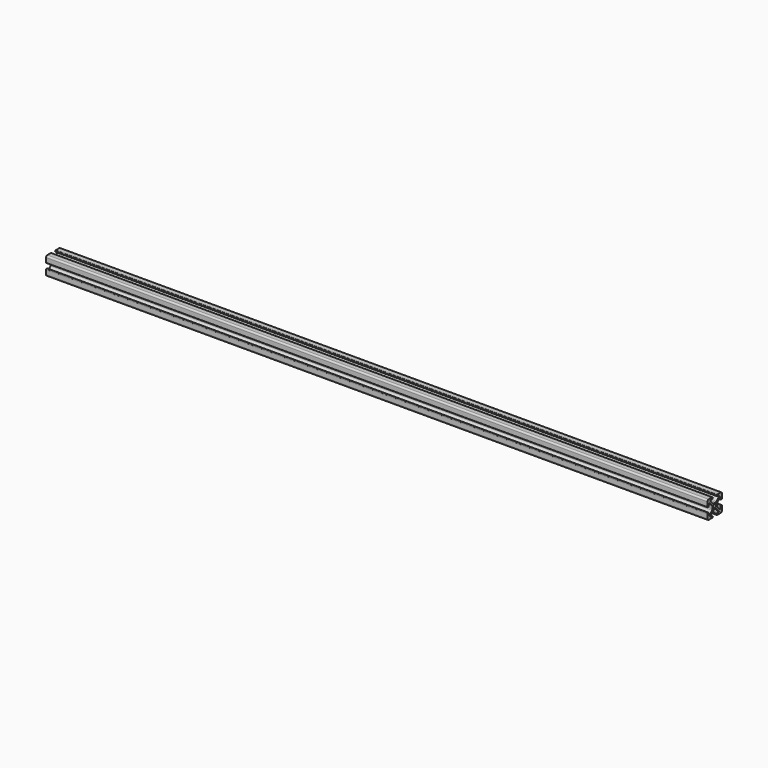
from build123d import *

# Parameters (mm, degrees)
F0_R     = 2.5
F2_DEPTH = 914.4
F3_R     = 2.14
F4_R     = 1.06999


# Not quite as in the source:
# - a fillet or chamfer is up to 0.001 mm smaller than in the source, because OpenCascade refuses the exact size


with BuildPart() as f2:
    # F0 (on Right) → F2 (new body)
    with BuildSketch(Plane.YZ):
        Polygon((2.5367914883, -4.05), (4.05, -4.05), (4.05, -2.5367914883), (4.05, 2.5367914883), (4.05, 4.05), (2.5367914883, 4.05), (-2.5367914883, 4.05), (-4.05, 4.05), (-4.05, 2.5367914883), (-4.05, -2.5367914883), (-4.05, -4.05), (-2.5367914883, -4.05), align=None)
        Circle(F0_R, mode=Mode.SUBTRACT)
        Polygon((-10.36, 8.8467914883), (-4.05, 2.5367914883), (-4.05, 4.05), (-2.5367914883, 4.05), (-8.8467914883, 10.36), (-3.25, 10.36), (-3.25, 12.5), (-12.5, 12.5), (-12.5, 3.25), (-10.36, 3.25), align=None)
        Polygon((4.05, 4.05), (4.05, 2.5367914883), (10.36, 8.8467914883), (10.36, 3.25), (12.5, 3.25), (12.5, 12.5), (3.25, 12.5), (3.25, 10.36), (8.8467914883, 10.36), (2.5367914883, 4.05), align=None)
        Polygon((-8.8467914883, -10.36), (-2.5367914883, -4.05), (-4.05, -4.05), (-4.05, -2.5367914883), (-10.36, -8.8467914883), (-10.36, -3.25), (-12.5, -3.25), (-12.5, -12.5), (-3.25, -12.5), (-3.25, -10.36), align=None)
        Polygon((4.05, -2.5367914883), (4.05, -4.05), (2.5367914883, -4.05), (8.8467914883, -10.36), (3.25, -10.36), (3.25, -12.5), (12.5, -12.5), (12.5, -3.25), (10.36, -3.25), (10.36, -8.8467914883), align=None)
    extrude(amount=F2_DEPTH)

    # F3
    f3_edges = [f2.edges().sort_by_distance(p)[0] for p in [
        (457.2, -12.5, 12.5),
        (457.2, 12.5, 12.5),
        (457.2, 12.5, -12.5),
        (457.2, -12.5, -12.5),
        (457.2, -4.05, 2.536791),
        (457.2, -4.05, -2.536791),
        (457.2, -2.536791, 4.05),
        (457.2, 2.536791, 4.05),
        (457.2, 4.05, 2.536791),
        (457.2, 4.05, -2.536791),
        (457.2, -2.536791, -4.05),
        (457.2, 2.536791, -4.05),
    ]]
    fillet(f3_edges, radius=F3_R)

    # F4 (radius 1.07 in the source; OpenCascade refuses exactly that, so slightly less here)
    f4_edges = [f2.edges().sort_by_distance(p)[0] for p in [
        (457.2, -12.5, 3.25),
        (457.2, -10.36, 3.25),
        (457.2, -3.25, 12.5),
        (457.2, -3.25, 10.36),
        (457.2, 3.25, 12.5),
        (457.2, 3.25, 10.36),
        (457.2, 10.36, 3.25),
        (457.2, 12.5, 3.25),
        (457.2, 10.36, -3.25),
        (457.2, 12.5, -3.25),
        (457.2, 3.25, -10.36),
        (457.2, 3.25, -12.5),
        (457.2, -3.25, -10.36),
        (457.2, -3.25, -12.5),
        (457.2, -10.36, 8.846791),
        (457.2, -8.846791, 10.36),
        (457.2, 8.846791, 10.36),
        (457.2, 10.36, 8.846791),
        (457.2, 8.846791, -10.36),
        (457.2, 10.36, -8.846791),
        (457.2, -8.846791, -10.36),
        (457.2, -10.36, -8.846791),
        (457.2, -10.36, -3.25),
        (457.2, -12.5, -3.25),
    ]]
    fillet(f4_edges, radius=F4_R)


solid = f2.part
